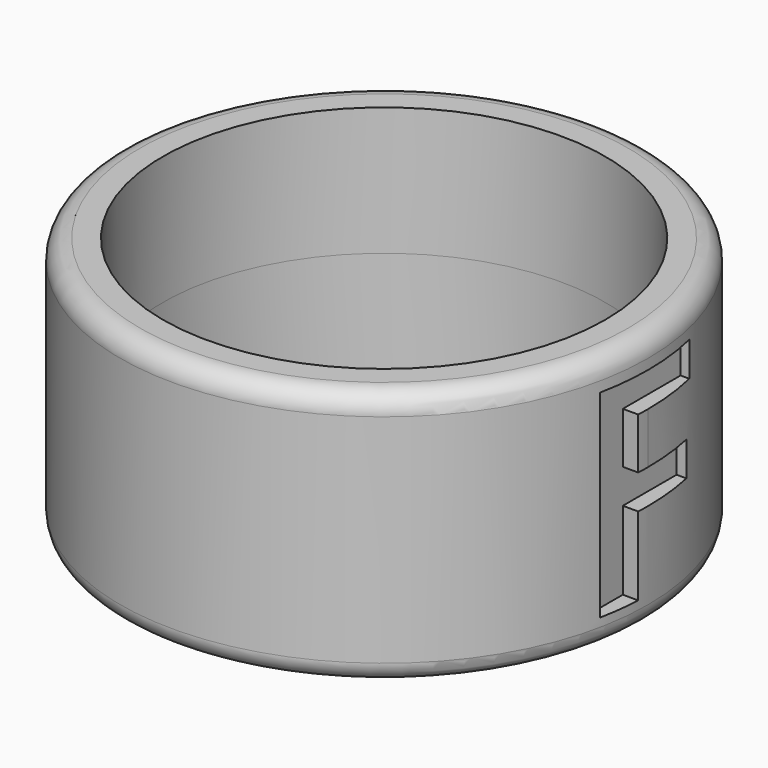
from build123d import *

# Parameters (mm, degrees)
F0_R          = 9.25
F0_R_2        = 7.75
F1_DEPTH      = 4.5
F1_DEPTH_BACK = 4.5
F2_R          = 0.7
F4_TEXT_SIZE  = 9.7222222222
F5_DEPTH      = 1.3


# Not quite as in the source:
# - Text() gives the source's letters only with a copy of the font that has no kerning and outlines rounded to 1/6400 em; it was checked with that copy


with BuildPart() as f1:
    # F0 (on Top) → F1 (new body, two sides)
    with BuildSketch(Plane.XY) as f1_sk:
        Circle(F0_R)
        Circle(F0_R_2, mode=Mode.SUBTRACT)
    extrude(amount=F1_DEPTH)
    extrude(f1_sk.sketch, amount=-F1_DEPTH_BACK)

    # F2
    f2_edges = [f1.edges().sort_by_distance(p)[0] for p in [
        (-9.25, 0, 4.5),
        (-9.25, 0, -4.5),
    ]]
    fillet(f2_edges, radius=F2_R)

    # F4 (on offset) → F5 (cut)
    with BuildSketch(Plane.YZ.offset(10)):
        with Locations((-2.7412109375, -3.5)):
            Text('F', F4_TEXT_SIZE, font='Open Sans', font_style=FontStyle.BOLD, text_align=(TextAlign.LEFT, TextAlign.BOTTOM))
    extrude(amount=-F5_DEPTH, mode=Mode.SUBTRACT)


solid = f1.part
